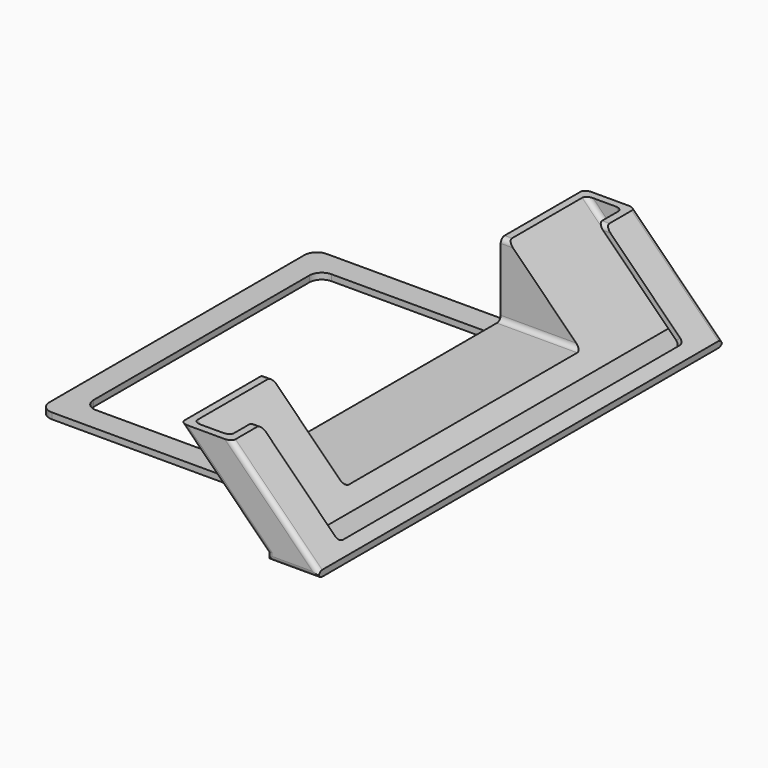
from build123d import *

# Parameters (mm, degrees)
F1_DEPTH      = 70
F2_DEPTH      = 103
F3_DEPTH      = 100
F4_W          = 175.6275002956
F4_H          = 18.8999543782
F4_H_2        = 45
F5_DEPTH      = 5
F6_DEPTH      = 70
F7_W          = 60.2522194386
F7_H          = 29.7944860623
F8_DEPTH      = 77
F9_W          = 73.7954185358
F9_H          = 120
F10_DEPTH     = 25
F11_R         = 5
F12_T1_DEPTH  = 2.1213203436
F12_T6_DEPTH  = 60
F12_T12_DEPTH = 60
F12_T18_DEPTH = 60
F12_T24_DEPTH = 60
F12_T30_DEPTH = 37.7944860623
F12_T35_DEPTH = 37.7944860623
F12_T37_DEPTH = 60
F12_T39_DEPTH = 13
F12_T41_DEPTH = 13
F12_T43_DEPTH = 30.8492424049
F12_T48_DEPTH = 60
F12_T53_DEPTH = 60
F12_T58_DEPTH = 12.5
F12_T63_DEPTH = 12.5
F12_T69_DEPTH = 7.5
F12_T73_DEPTH = 60
F12_T81_DEPTH = 7.5
F12_T85_DEPTH = 60


# Not quite as in the source:
# - a fillet or chamfer that OpenCascade refuses, or shapes differently, is made with other operations: its cross-section is extruded or revolved along the edge and cut away or added


with BuildPart() as f1:
    # F0 (on Front) → F1 (new body, symmetric)
    with BuildSketch(Plane.XZ):
        Polygon((-140, 0), (-20.8492424049, 0), (-20.8492424049, 2.5), (-53.2045814642, 2.5), (-56.2045814642, 2.5), (-140, 2.5), align=None)
    extrude(amount=F1_DEPTH, both=True)

    # F0 (on Front) → F2 (join, symmetric)
    with BuildSketch(Plane.XZ):
        Polygon((-20.8492424049, 0), (0, 0), (0, 2.5), (-3, 2.5), (-17.8492424049, 2.5), (-20.8492424049, 2.5), align=None)
        Polygon((-53.2045814642, 34.8553390593), (-20.8492424049, 2.5), (-17.8492424049, 2.5), (-53.2045814642, 37.8553390593), (-56.2045814642, 37.8553390593), align=None)
        Polygon((-3, 2.5), (0, 2.5), (-35.3553390593, 37.8553390593), (-38.3553390593, 37.8553390593), align=None)
        Polygon((-17.8492424049, 2.5), (-3, 2.5), (-38.3553390593, 37.8553390593), (-53.2045814642, 37.8553390593), align=None)
    extrude(amount=F2_DEPTH, both=True)

    # F0 (on Front) → F3 (cut, symmetric)
    with BuildSketch(Plane.XZ):
        Polygon((-17.8492424049, 2.5), (-3, 2.5), (-38.3553390593, 37.8553390593), (-53.2045814642, 37.8553390593), align=None)
    extrude(amount=F3_DEPTH, both=True, mode=Mode.SUBTRACT)

    # F4 (on face) → F5 (cut)
    with BuildSketch(Plane(origin=(1.25, 0, 1.25), x_dir=(0, 1, 0), z_dir=(0.7071067812, 0, 0.7071067812))):
        with Locations((-0.1862498522, 61.217744142)):
            Rectangle(F4_W, F4_H)
        with Locations((-0.1862498522, 29.267766953)):
            Rectangle(F4_W, F4_H_2)
    extrude(amount=-F5_DEPTH, mode=Mode.SUBTRACT)

    # F0 (on Front) → F6 (join, symmetric)
    with BuildSketch(Plane.XZ):
        Polygon((-53.2045814642, 2.5), (-20.8492424049, 2.5), (-53.2045814642, 34.8553390593), align=None)
        Polygon((-56.2045814642, 2.5), (-53.2045814642, 2.5), (-53.2045814642, 34.8553390593), (-56.2045814642, 37.8553390593), align=None)
    extrude(amount=F6_DEPTH, both=True)

    # F7 (on face) → F8 (cut)
    with BuildSketch(Plane(origin=(-56.2045814642, 0, 0), x_dir=(0, -1, 0), z_dir=(-1, 0, 0))):
        with Locations((-30.1261097193, 22.9580960282)):
            Rectangle(F7_W, F7_H)
        with Locations((30.1261097193, 22.9580960282)):
            Rectangle(F7_W, F7_H)
    extrude(amount=-F8_DEPTH, mode=Mode.SUBTRACT)

    # F9 (on face) → F10 (cut)
    with BuildSketch(Plane.XY.offset(2.5)):
        with Locations((-93.1022907321, 0)):
            Rectangle(F9_W, F9_H)
    extrude(amount=-F10_DEPTH, mode=Mode.SUBTRACT)

    # F11
    f11_edges = [f1.edges().sort_by_distance(p)[0] for p in [
        (-56.204581, 65, 2.5),
        (-56.204581, -65, 2.5),
        (-140, -70, 1.25),
        (-140, 70, 1.25),
        (-130, -60, 1.25),
        (-130, 60, 1.25),
        (-56.204581, 60, 1.25),
        (-56.204581, -60, 1.25),
    ]]
    fillet(f11_edges, radius=F11_R)

    # F12: fillet of radius 2 on 20 edges, made by hand

    # F12_s2 → F12_t1 (join)
    with BuildSketch(Plane(origin=(1.25, 0, 1.25), x_dir=(0, 1, 0), z_dir=(-0.7071067812, 0, -0.7071067812))):
        with BuildLine():
            ThreePointArc((87.6275002956, -8.767766953), (87.041713858, -7.3535533906), (85.6275002956, -6.767766953))
            Line((85.6275002956, -6.767766953), (87.6275002956, -6.767766953))
            Line((87.6275002956, -6.767766953), (87.6275002956, -8.767766953))
        make_face()
        with BuildLine():
            ThreePointArc((-88, -8.767766953), (-87.4142135624, -7.3535533906), (-86, -6.767766953))
            Line((-86, -6.767766953), (-88, -6.767766953))
            Line((-88, -6.767766953), (-88, -8.767766953))
        make_face()
    extrude(amount=F12_T1_DEPTH)


with BuildPart() as f12_tool4:
    # F12_s5 → F12_t6 (new body)
    with BuildSketch(Plane(origin=(0.7855339059, 0, -0.7855339059), x_dir=(0, 1, 0), z_dir=(-0.7071067812, 0, 0.7071067812))):
        with BuildLine():
            ThreePointArc((-98, 0.3535533906), (-99.4142135624, 0.9393398282), (-100, 2.3535533906))
            Line((-100, 2.3535533906), (-100, 0.3535533906))
            Line((-100, 0.3535533906), (-98, 0.3535533906))
        make_face()
    extrude(amount=F12_T6_DEPTH)

    split(bisect_by=Plane.XY.offset(37.8553390593), keep=Keep.BOTTOM)

    split(bisect_by=Plane.XY.offset(2.5), keep=Keep.TOP)


with BuildPart() as f1_1:
    add(f1.part)

    # F12_t3: union F12_tool4
    add(f12_tool4.part)


with BuildPart() as f12_tool10:
    # F12_s11 → F12_t12 (new body)
    with BuildSketch(Plane(origin=(-49.0654941677, 0, 49.0654941677), x_dir=(0, 1, 0), z_dir=(0.7071067812, 0, -0.7071067812))):
        with BuildLine():
            ThreePointArc((-98, -10.8535533906), (-99.4142135624, -10.267766953), (-100, -8.8535533906))
            Line((-100, -8.8535533906), (-100, -10.8535533906))
            Line((-100, -10.8535533906), (-98, -10.8535533906))
        make_face()
    extrude(amount=F12_T12_DEPTH)

    split(bisect_by=Plane.XY.offset(37.8553390593), keep=Keep.BOTTOM)

    split(bisect_by=Plane.XY.offset(2.5), keep=Keep.TOP)


with BuildPart() as f1_2:
    add(f1_1.part)

    # F12_t9: union F12_tool10
    add(f12_tool10.part)


with BuildPart() as f12_tool16:
    # F12_s17 → F12_t18 (new body)
    with BuildSketch(Plane(origin=(-49.0654941677, 0, 49.0654941677), x_dir=(0, 1, 0), z_dir=(0.7071067812, 0, -0.7071067812))):
        with BuildLine():
            ThreePointArc((100, -8.8535533906), (99.4142135624, -10.267766953), (98, -10.8535533906))
            Line((98, -10.8535533906), (100, -10.8535533906))
            Line((100, -10.8535533906), (100, -8.8535533906))
        make_face()
    extrude(amount=F12_T18_DEPTH)

    split(bisect_by=Plane.XY.offset(37.8553390593), keep=Keep.BOTTOM)

    split(bisect_by=Plane.XY.offset(2.5), keep=Keep.TOP)


with BuildPart() as f1_3:
    add(f1_2.part)

    # F12_t15: union F12_tool16
    add(f12_tool16.part)


with BuildPart() as f12_tool22:
    # F12_s23 → F12_t24 (new body)
    with BuildSketch(Plane(origin=(0.7855339059, 0, -0.7855339059), x_dir=(0, 1, 0), z_dir=(-0.7071067812, 0, 0.7071067812))):
        with BuildLine():
            ThreePointArc((98, 0.3535533906), (99.4142135624, 0.9393398282), (100, 2.3535533906))
            Line((100, 2.3535533906), (100, 0.3535533906))
            Line((100, 0.3535533906), (98, 0.3535533906))
        make_face()
    extrude(amount=F12_T24_DEPTH)

    split(bisect_by=Plane.XY.offset(37.8553390593), keep=Keep.BOTTOM)

    split(bisect_by=Plane.XY.offset(2.5), keep=Keep.TOP)


with BuildPart() as f1_4:
    add(f1_3.part)

    # F12_t21: union F12_tool22
    add(f12_tool22.part)


with BuildPart() as f12_tool28:
    # F12_s29 → F12_t30 (new body)
    with BuildSketch(Plane.YZ.offset(-56.2045814642)):
        with BuildLine():
            ThreePointArc((-58.2522194386, 8.060852997), (-59.6664330009, 8.6466394346), (-60.2522194386, 10.060852997))
            Line((-60.2522194386, 10.060852997), (-60.2522194386, 8.060852997))
            Line((-60.2522194386, 8.060852997), (-58.2522194386, 8.060852997))
        make_face()
    extrude(amount=F12_T30_DEPTH)

    split(bisect_by=Plane(origin=(-7.6746212025, 0, -7.6746212025), x_dir=(0, 1, 0), z_dir=(-0.7071067812, 0, -0.7071067812)), keep=Keep.TOP)


with BuildPart() as f1_5:
    add(f1_4.part)

    # F12_t27: union F12_tool28
    add(f12_tool28.part)


with BuildPart() as f12_tool33:
    # F12_s34 → F12_t35 (new body)
    with BuildSketch(Plane.YZ.offset(-56.2045814642)):
        with BuildLine():
            ThreePointArc((60.2522194386, 10.060852997), (59.6664330009, 8.6466394346), (58.2522194386, 8.060852997))
            Line((58.2522194386, 8.060852997), (60.2522194386, 8.060852997))
            Line((60.2522194386, 8.060852997), (60.2522194386, 10.060852997))
        make_face()
    extrude(amount=F12_T35_DEPTH)

    split(bisect_by=Plane(origin=(-7.6746212025, 0, -7.6746212025), x_dir=(0, 1, 0), z_dir=(-0.7071067812, 0, -0.7071067812)), keep=Keep.TOP)


with BuildPart() as f1_6:
    add(f1_5.part)

    # F12_t32: union F12_tool33
    add(f12_tool33.part)

    # F12_s38 → F12_t37 (cut)
    with BuildSketch(Plane(origin=(2.2855339059, 0, -2.2855339059), x_dir=(0, 1, 0), z_dir=(-0.7071067812, 0, 0.7071067812))):
        with BuildLine():
            ThreePointArc((-103, 0.232233047), (-102.4142135624, -1.1819805153), (-101, -1.767766953))
            Line((-101, -1.767766953), (-103, -1.767766953))
            Line((-103, -1.767766953), (-103, 0.232233047))
        make_face()
        with BuildLine():
            ThreePointArc((103, 0.232233047), (102.4142135624, -1.1819805153), (101, -1.767766953))
            Line((101, -1.767766953), (103, -1.767766953))
            Line((103, -1.767766953), (103, 0.232233047))
        make_face()
    extrude(amount=F12_T37_DEPTH, mode=Mode.SUBTRACT)

    # F12_s40 → F12_t39 (cut)
    with BuildSketch(Plane.YZ.offset(-43.3553390593)):
        with BuildLine():
            ThreePointArc((-90, 37.8553390593), (-88.5857864376, 37.2695526217), (-88, 35.8553390593))
            Line((-88, 35.8553390593), (-88, 37.8553390593))
            Line((-88, 37.8553390593), (-90, 37.8553390593))
        make_face()
        with BuildLine():
            ThreePointArc((89.6275002956, 37.8553390593), (88.2132867333, 37.2695526217), (87.6275002956, 35.8553390593))
            Line((87.6275002956, 35.8553390593), (87.6275002956, 37.8553390593))
            Line((87.6275002956, 37.8553390593), (89.6275002956, 37.8553390593))
        make_face()
    extrude(amount=F12_T39_DEPTH, mode=Mode.SUBTRACT)

    # F12_s42 → F12_t41 (cut)
    with BuildSketch(Plane.YZ.offset(-61.2045814642)):
        with BuildLine():
            ThreePointArc((62.2522194386, 37.8553390593), (60.8380058762, 37.2695526217), (60.2522194386, 35.8553390593))
            Line((60.2522194386, 35.8553390593), (60.2522194386, 37.8553390593))
            Line((60.2522194386, 37.8553390593), (62.2522194386, 37.8553390593))
        make_face()
        with BuildLine():
            ThreePointArc((-60.2522194386, 35.8553390593), (-60.8380058762, 37.2695526217), (-62.2522194386, 37.8553390593))
            Line((-62.2522194386, 37.8553390593), (-60.2522194386, 37.8553390593))
            Line((-60.2522194386, 37.8553390593), (-60.2522194386, 35.8553390593))
        make_face()
    extrude(amount=F12_T41_DEPTH, mode=Mode.SUBTRACT)

    # F12_s44 → F12_t43 (cut)
    with BuildSketch(Plane.YZ.offset(-25.8492424049)):
        with BuildLine():
            ThreePointArc((-101, 0), (-102.4142135624, 0.5857864376), (-103, 2))
            Line((-103, 2), (-103, 0))
            Line((-103, 0), (-101, 0))
        make_face()
        with BuildLine():
            ThreePointArc((101, 0), (102.4142135624, 0.5857864376), (103, 2))
            Line((103, 2), (103, 0))
            Line((103, 0), (101, 0))
        make_face()
    extrude(amount=F12_T43_DEPTH, mode=Mode.SUBTRACT)


with BuildPart() as f12_tool46:
    # F12_s47 → F12_t48 (new body)
    with BuildSketch(Plane(origin=(-50.5654941677, 0, 50.5654941677), x_dir=(0, 1, 0), z_dir=(0.7071067812, 0, -0.7071067812))):
        with BuildLine():
            ThreePointArc((-103, -10.9748737342), (-102.4142135624, -12.3890872965), (-101, -12.9748737342))
            Line((-101, -12.9748737342), (-103, -12.9748737342))
            Line((-103, -12.9748737342), (-103, -10.9748737342))
        make_face()
    extrude(amount=F12_T48_DEPTH)

    split(bisect_by=Plane.YZ.offset(-20.8492424049), keep=Keep.BOTTOM)


with BuildPart() as f1_7:
    add(f1_6.part)

    # F12_t45: cut F12_tool46
    add(f12_tool46.part, mode=Mode.SUBTRACT)


with BuildPart() as f12_tool51:
    # F12_s52 → F12_t53 (new body)
    with BuildSketch(Plane(origin=(-50.5654941677, 0, 50.5654941677), x_dir=(0, 1, 0), z_dir=(0.7071067812, 0, -0.7071067812))):
        with BuildLine():
            ThreePointArc((101, -12.9748737342), (102.4142135624, -12.3890872965), (103, -10.9748737342))
            Line((103, -10.9748737342), (103, -12.9748737342))
            Line((103, -12.9748737342), (101, -12.9748737342))
        make_face()
    extrude(amount=F12_T53_DEPTH)

    split(bisect_by=Plane.YZ.offset(-20.8492424049), keep=Keep.BOTTOM)


with BuildPart() as f1_8:
    add(f1_7.part)

    # F12_t50: cut F12_tool51
    add(f12_tool51.part, mode=Mode.SUBTRACT)


with BuildPart() as f12_tool56:
    # F12_s57 → F12_t58 (new body)
    with BuildSketch(Plane.XY.offset(7.5)):
        with BuildLine():
            ThreePointArc((-20.8492424049, 101), (-20.2634559673, 102.4142135624), (-18.8492424049, 103))
            Line((-18.8492424049, 103), (-20.8492424049, 103))
            Line((-20.8492424049, 103), (-20.8492424049, 101))
        make_face()
    extrude(amount=-F12_T58_DEPTH)

    split(bisect_by=Plane(origin=(-9.1746212025, 0, -9.1746212025), x_dir=(0, 1, 0), z_dir=(-0.7071067812, 0, -0.7071067812)), keep=Keep.TOP)


with BuildPart() as f1_9:
    add(f1_8.part)

    # F12_t55: cut F12_tool56
    add(f12_tool56.part, mode=Mode.SUBTRACT)


with BuildPart() as f12_tool61:
    # F12_s62 → F12_t63 (new body)
    with BuildSketch(Plane.XY.offset(7.5)):
        with BuildLine():
            ThreePointArc((-18.8492424049, -103), (-20.2634559673, -102.4142135624), (-20.8492424049, -101))
            Line((-20.8492424049, -101), (-20.8492424049, -103))
            Line((-20.8492424049, -103), (-18.8492424049, -103))
        make_face()
    extrude(amount=-F12_T63_DEPTH)

    split(bisect_by=Plane(origin=(-9.1746212025, 0, -9.1746212025), x_dir=(0, 1, 0), z_dir=(-0.7071067812, 0, -0.7071067812)), keep=Keep.TOP)


with BuildPart() as f1_10:
    add(f1_9.part)

    # F12_t60: cut F12_tool61
    add(f12_tool61.part, mode=Mode.SUBTRACT)


with BuildPart() as f12_tool67:
    # F12_s68 → F12_t69 (new body)
    with BuildSketch(Plane.XY.offset(7.5)):
        with BuildLine():
            ThreePointArc((-18.8492424049, -103), (-20.2634559673, -102.4142135624), (-20.8492424049, -101))
            Line((-20.8492424049, -101), (-20.8492424049, -103))
            Line((-20.8492424049, -103), (-18.8492424049, -103))
        make_face()
    extrude(amount=-F12_T69_DEPTH)

    split(bisect_by=Plane(origin=(-9.1746212025, 0, -9.1746212025), x_dir=(0, 1, 0), z_dir=(0.7071067812, 0, 0.7071067812)), keep=Keep.TOP)


with BuildPart() as f12_tool71:
    # F12_s72 → F12_t73 (new body)
    with BuildSketch(Plane(origin=(-50.5654941677, 0, 50.5654941677), x_dir=(0, 1, 0), z_dir=(0.7071067812, 0, -0.7071067812))):
        with BuildLine():
            ThreePointArc((-103, -10.9748737342), (-102.4142135624, -12.3890872965), (-101, -12.9748737342))
            Line((-101, -12.9748737342), (-103, -12.9748737342))
            Line((-103, -12.9748737342), (-103, -10.9748737342))
        make_face()
    extrude(amount=F12_T73_DEPTH)

    split(bisect_by=Plane.XY, keep=Keep.TOP)

    split(bisect_by=Plane.YZ.offset(-20.8492424049), keep=Keep.TOP)


with BuildPart() as f12_tool67_1:
    add(f12_tool67.part)

    # F12_t76: intersect F12_tool71
    add(f12_tool71.part, mode=Mode.INTERSECT)


with BuildPart() as f1_11:
    add(f1_10.part)

    # F12_t65: cut F12_tool67
    add(f12_tool67_1.part, mode=Mode.SUBTRACT)


with BuildPart() as f12_tool79:
    # F12_s80 → F12_t81 (new body)
    with BuildSketch(Plane.XY.offset(7.5)):
        with BuildLine():
            ThreePointArc((-20.8492424049, 101), (-20.2634559673, 102.4142135624), (-18.8492424049, 103))
            Line((-18.8492424049, 103), (-20.8492424049, 103))
            Line((-20.8492424049, 103), (-20.8492424049, 101))
        make_face()
    extrude(amount=-F12_T81_DEPTH)

    split(bisect_by=Plane(origin=(-9.1746212025, 0, -9.1746212025), x_dir=(0, 1, 0), z_dir=(0.7071067812, 0, 0.7071067812)), keep=Keep.TOP)


with BuildPart() as f12_tool83:
    # F12_s84 → F12_t85 (new body)
    with BuildSketch(Plane(origin=(-50.5654941677, 0, 50.5654941677), x_dir=(0, 1, 0), z_dir=(0.7071067812, 0, -0.7071067812))):
        with BuildLine():
            ThreePointArc((101, -12.9748737342), (102.4142135624, -12.3890872965), (103, -10.9748737342))
            Line((103, -10.9748737342), (103, -12.9748737342))
            Line((103, -12.9748737342), (101, -12.9748737342))
        make_face()
    extrude(amount=F12_T85_DEPTH)

    split(bisect_by=Plane.XY, keep=Keep.TOP)

    split(bisect_by=Plane.YZ.offset(-20.8492424049), keep=Keep.TOP)


with BuildPart() as f12_tool79_1:
    add(f12_tool79.part)

    # F12_t88: intersect F12_tool83
    add(f12_tool83.part, mode=Mode.INTERSECT)


with BuildPart() as f1_12:
    add(f1_11.part)

    # F12_t77: cut F12_tool79
    add(f12_tool79_1.part, mode=Mode.SUBTRACT)


solid = f1_12.part
